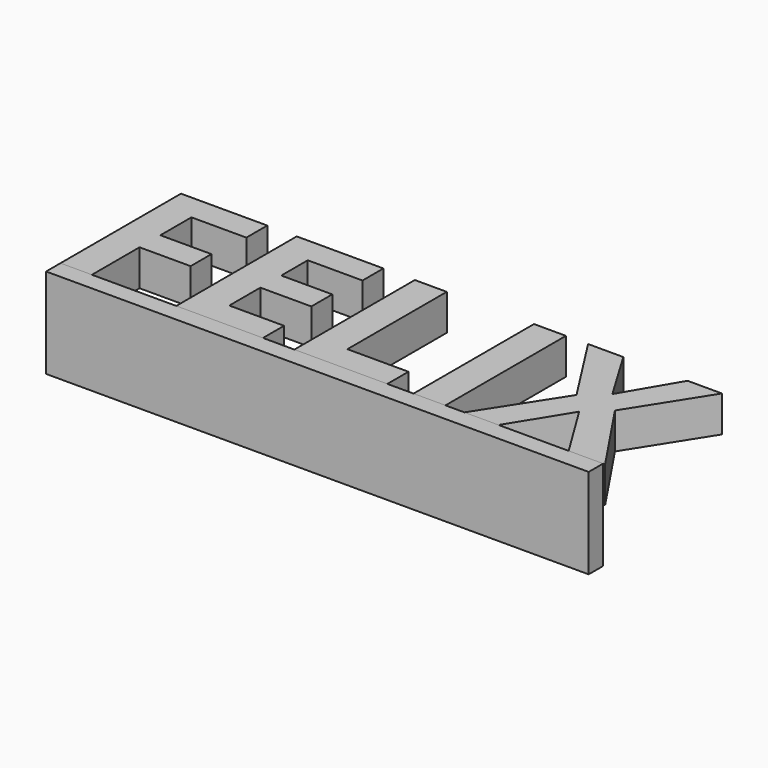
from build123d import *

# Parameters (mm, degrees)
F0_TEXT_SIZE = 58.4608358073
F1_DEPTH     = 10
F2_W         = 150.4032468255
F2_H         = 25
F3_DEPTH     = 5


# Not quite as in the source:
# - Text() gives the source's letters only with a copy of the font that has no kerning and outlines rounded to 1/6400 em; it was checked with that copy


with BuildPart() as f1:
    # F0 (on Top) → F1 (new body)
    with BuildSketch(Plane.XY):
        with Locations((-78.4815905822, -18.3473665532)):
            Text('FELIX', F0_TEXT_SIZE, font='Open Sans', font_style=FontStyle.BOLD, text_align=(TextAlign.LEFT, TextAlign.BOTTOM))
    extrude(amount=F1_DEPTH)


with BuildPart() as f3:
    # F2 (on face) → F3 (new body)
    with BuildSketch(Plane.XZ.offset(18.3473665532)):
        with Locations((1.9723735476, -2.5)):
            Rectangle(F2_W, F2_H)
    extrude(amount=F3_DEPTH)


solid = Compound([f1.part, f3.part])
